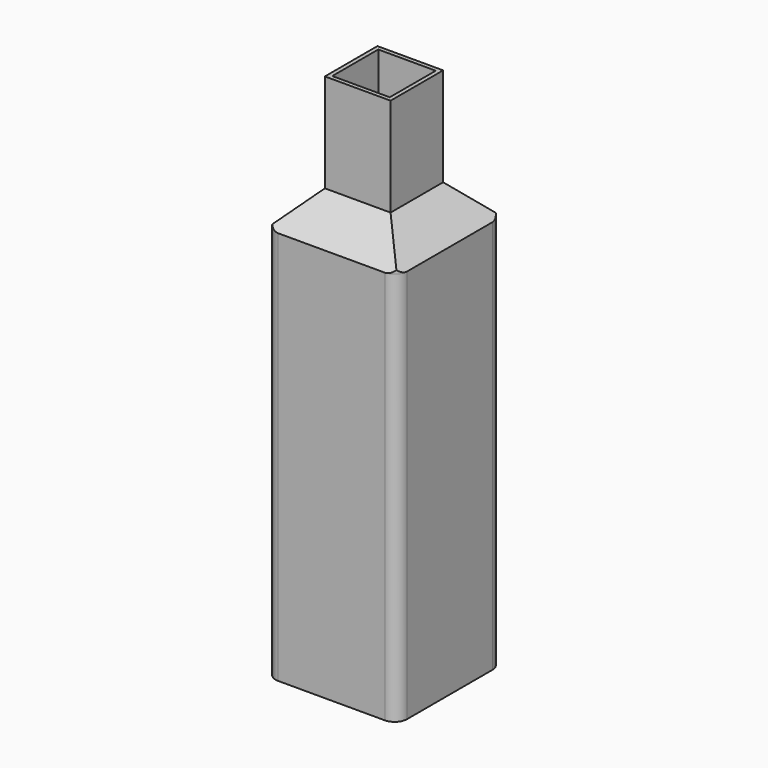
from build123d import *

# Parameters (mm, degrees)
F0_W         = 41.275
F0_H         = 41.275
F1_DEPTH     = 152.4
F3_W         = 41.275
F3_H         = 41.275
F4_DEPTH     = 25.4
F5_T1_DEPTH  = 171.9164957887
F5_T3_DEPTH  = 171.9164957887
F5_T8_ANGLE  = 90
F5_T13_ANGLE = 90
F5_T18_ANGLE = 90
F5_T23_ANGLE = 90
F5_T28_ANGLE = 90
F5_T33_ANGLE = 90
F5_T38_ANGLE = 90
F5_T43_ANGLE = 90
F2_W         = 25.4
F2_H         = 25.4
F2_W_2       = 22.225
F2_H_2       = 22.225
F6_DEPTH     = 203.2


# Not quite as in the source:
# - a fillet or chamfer that OpenCascade refuses, or shapes differently, is made with other operations: its cross-section is extruded or revolved along the edge and cut away or added


with BuildPart() as f1:
    # F0 (on Top) → F1 (new body)
    with BuildSketch(Plane.XY):
        with BuildLine():
            ThreePointArc((0, 4.7625), (1.3949039546, 1.3949039546), (4.7625, 0))
            Line((4.7625, 0), (46.0375, 0))
            ThreePointArc((46.0375, 0), (49.4050960454, 1.3949039546), (50.8, 4.7625))
            Line((50.8, 4.7625), (50.8, 46.0375))
            ThreePointArc((50.8, 46.0375), (49.4050960454, 49.4050960454), (46.0375, 50.8))
            Line((46.0375, 50.8), (4.7625, 50.8))
            ThreePointArc((4.7625, 50.8), (1.3949039546, 49.4050960454), (0, 46.0375))
            Line((0, 46.0375), (0, 4.7625))
        make_face()
        with Locations((25.4, 25.4)):
            Rectangle(F0_W, F0_H, mode=Mode.SUBTRACT)
    extrude(amount=F1_DEPTH)


with BuildPart() as f4:
    # F3 (on face) → F4 (new body)
    with BuildSketch(Plane.XY.offset(152.4)):
        with BuildLine():
            ThreePointArc((0, 4.7625), (1.3949039546, 1.3949039546), (4.7625, 0))
            Line((4.7625, 0), (46.0375, 0))
            ThreePointArc((46.0375, 0), (49.4050960454, 1.3949039546), (50.8, 4.7625))
            Line((50.8, 4.7625), (50.8, 46.0375))
            ThreePointArc((50.8, 46.0375), (49.4050960454, 49.4050960454), (46.0375, 50.8))
            Line((46.0375, 50.8), (4.7625, 50.8))
            ThreePointArc((4.7625, 50.8), (1.3949039546, 49.4050960454), (0, 46.0375))
            Line((0, 46.0375), (0, 4.7625))
        make_face()
        with Locations((25.4, 25.4)):
            Rectangle(F3_W, F3_H, mode=Mode.SUBTRACT)
        with Locations((25.4, 25.4)):
            Rectangle(F3_W, F3_H)
    extrude(amount=F4_DEPTH)

    # F5: chamfer of 25.4 on 4 edges, made by hand

    # F5_s2 → F5_t1 (cut)
    with BuildSketch(Plane.XZ.offset(-111.3582478943)):
        Polygon((50.8, 152.4), (25.4, 177.8), (50.8, 177.8), align=None)
        Polygon((0, 152.4), (25.4, 177.8), (0, 177.8), align=None)
    extrude(amount=F5_T1_DEPTH, mode=Mode.SUBTRACT)

    # F5_s4 → F5_t3 (cut)
    with BuildSketch(Plane.YZ.offset(-60.5582478943)):
        Polygon((50.8, 152.4), (25.4, 177.8), (50.8, 177.8), align=None)
        Polygon((0, 152.4), (25.4, 177.8), (0, 177.8), align=None)
    extrude(amount=F5_T3_DEPTH, mode=Mode.SUBTRACT)


with BuildPart() as f5_tool6:
    # F5_s7 → F5_t8 (revolve)
    with BuildSketch(Plane.YZ.offset(4.7625)):
        Polygon((50.8, 152.4), (46.0375, 157.1625), (46.0375, 177.8), (50.8, 177.8), align=None)
    revolve(axis=Axis((4.7625, 46.0375, 177.8), (0, 0, 1)), revolution_arc=F5_T8_ANGLE)

    split(bisect_by=Plane(origin=(0, 101.6, 101.6), x_dir=(1, 0, 0), z_dir=(0, 0.7071067812, 0.7071067812)), keep=Keep.TOP)


with BuildPart() as f4_1:
    add(f4.part)

    # F5_t5: cut F5_tool6
    add(f5_tool6.part, mode=Mode.SUBTRACT)


with BuildPart() as f5_tool11:
    # F5_s12 → F5_t13 (revolve)
    with BuildSketch(Plane.YZ.offset(4.7625)):
        Polygon((50.8, 152.4), (46.0375, 157.1625), (46.0375, 177.8), (50.8, 177.8), align=None)
    revolve(axis=Axis((4.7625, 46.0375, 177.8), (0, 0, 1)), revolution_arc=F5_T13_ANGLE)

    split(bisect_by=Plane(origin=(-76.2, 0, 76.2), x_dir=(0, 1, 0), z_dir=(-0.7071067812, 0, 0.7071067812)), keep=Keep.TOP)


with BuildPart() as f4_2:
    add(f4_1.part)

    # F5_t10: cut F5_tool11
    add(f5_tool11.part, mode=Mode.SUBTRACT)


with BuildPart() as f5_tool16:
    # F5_s17 → F5_t18 (revolve)
    with BuildSketch(Plane.XZ.offset(-4.7625)):
        Polygon((0, 152.4), (4.7625, 157.1625), (4.7625, 177.8), (0, 177.8), align=None)
    revolve(axis=Axis((4.7625, 4.7625, 177.8), (0, 0, 1)), revolution_arc=F5_T18_ANGLE)

    split(bisect_by=Plane(origin=(-76.2, 0, 76.2), x_dir=(0, 1, 0), z_dir=(-0.7071067812, 0, 0.7071067812)), keep=Keep.TOP)


with BuildPart() as f4_3:
    add(f4_2.part)

    # F5_t15: cut F5_tool16
    add(f5_tool16.part, mode=Mode.SUBTRACT)


with BuildPart() as f5_tool21:
    # F5_s22 → F5_t23 (revolve)
    with BuildSketch(Plane.XZ.offset(-4.7625)):
        Polygon((0, 152.4), (4.7625, 157.1625), (4.7625, 177.8), (0, 177.8), align=None)
    revolve(axis=Axis((4.7625, 4.7625, 177.8), (0, 0, 1)), revolution_arc=F5_T23_ANGLE)

    split(bisect_by=Plane(origin=(0, -76.2, 76.2), x_dir=(1, 0, 0), z_dir=(0, -0.7071067812, 0.7071067812)), keep=Keep.TOP)


with BuildPart() as f4_4:
    add(f4_3.part)

    # F5_t20: cut F5_tool21
    add(f5_tool21.part, mode=Mode.SUBTRACT)


with BuildPart() as f5_tool26:
    # F5_s27 → F5_t28 (revolve)
    with BuildSketch(Plane.YZ.offset(46.0375)):
        Polygon((0, 152.4), (4.7625, 157.1625), (4.7625, 177.8), (0, 177.8), align=None)
    revolve(axis=Axis((46.0375, 4.7625, 177.8), (0, 0, 1)), revolution_arc=F5_T28_ANGLE)

    split(bisect_by=Plane(origin=(0, -76.2, 76.2), x_dir=(1, 0, 0), z_dir=(0, -0.7071067812, 0.7071067812)), keep=Keep.TOP)


with BuildPart() as f4_5:
    add(f4_4.part)

    # F5_t25: cut F5_tool26
    add(f5_tool26.part, mode=Mode.SUBTRACT)


with BuildPart() as f5_tool31:
    # F5_s32 → F5_t33 (revolve)
    with BuildSketch(Plane.YZ.offset(46.0375)):
        Polygon((0, 152.4), (4.7625, 157.1625), (4.7625, 177.8), (0, 177.8), align=None)
    revolve(axis=Axis((46.0375, 4.7625, 177.8), (0, 0, 1)), revolution_arc=F5_T33_ANGLE)

    split(bisect_by=Plane(origin=(101.6, 0, 101.6), x_dir=(0, 1, 0), z_dir=(0.7071067812, 0, 0.7071067812)), keep=Keep.TOP)


with BuildPart() as f4_6:
    add(f4_5.part)

    # F5_t30: cut F5_tool31
    add(f5_tool31.part, mode=Mode.SUBTRACT)


with BuildPart() as f5_tool36:
    # F5_s37 → F5_t38 (revolve)
    with BuildSketch(Plane.XZ.offset(-46.0375)):
        Polygon((50.8, 152.4), (46.0375, 157.1625), (46.0375, 177.8), (50.8, 177.8), align=None)
    revolve(axis=Axis((46.0375, 46.0375, 177.8), (0, 0, 1)), revolution_arc=F5_T38_ANGLE)

    split(bisect_by=Plane(origin=(101.6, 0, 101.6), x_dir=(0, 1, 0), z_dir=(0.7071067812, 0, 0.7071067812)), keep=Keep.TOP)


with BuildPart() as f4_7:
    add(f4_6.part)

    # F5_t35: cut F5_tool36
    add(f5_tool36.part, mode=Mode.SUBTRACT)


with BuildPart() as f5_tool41:
    # F5_s42 → F5_t43 (revolve)
    with BuildSketch(Plane.XZ.offset(-46.0375)):
        Polygon((50.8, 152.4), (46.0375, 157.1625), (46.0375, 177.8), (50.8, 177.8), align=None)
    revolve(axis=Axis((46.0375, 46.0375, 177.8), (0, 0, 1)), revolution_arc=F5_T43_ANGLE)

    split(bisect_by=Plane(origin=(0, 101.6, 101.6), x_dir=(1, 0, 0), z_dir=(0, 0.7071067812, 0.7071067812)), keep=Keep.TOP)


with BuildPart() as f4_8:
    add(f4_7.part)

    # F5_t40: cut F5_tool41
    add(f5_tool41.part, mode=Mode.SUBTRACT)


with BuildPart() as f6:
    # F2 (on Top) → F6 (new body)
    with BuildSketch(Plane.XY):
        with Locations((25.4, 25.4)):
            Rectangle(F2_W, F2_H)
        with Locations((25.4, 25.4)):
            Rectangle(F2_W_2, F2_H_2, mode=Mode.SUBTRACT)
    extrude(amount=F6_DEPTH)


solid = Compound([f1.part, f4_8.part, f6.part])
